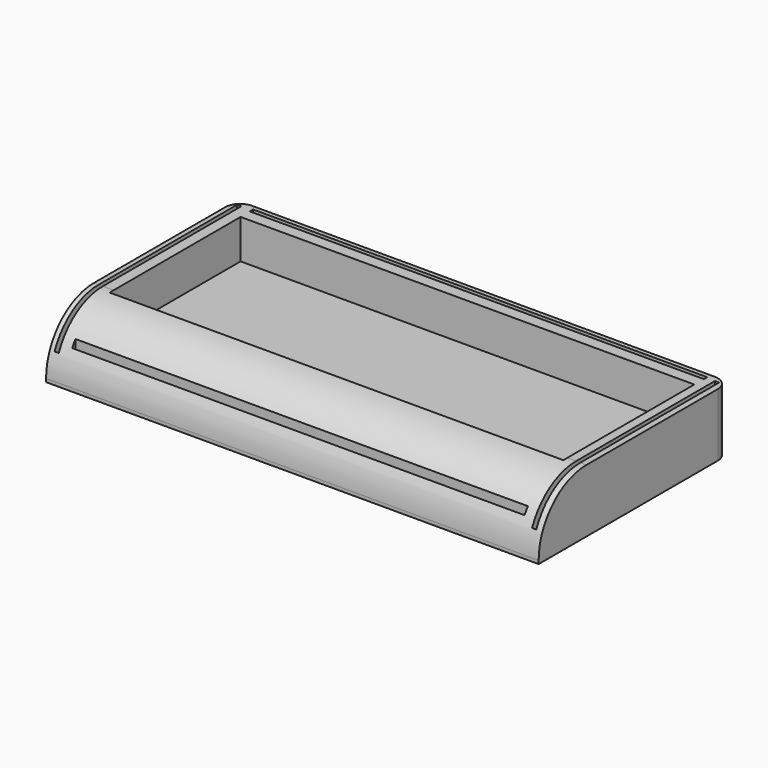
from build123d import *

# Parameters (mm, degrees)
F0_W        = 165
F0_H        = 80
F0_W_2      = 151.5524461865
F0_H_2      = 1.4
F0_W_3      = 1.4
F0_H_3      = 76.4191485941
F0_H_4      = 76.5563435853
F0_W_4      = 151.9825384021
F0_H_5      = 54.7616053373
F0_W_5      = 152.1170958877
F1_DEPTH    = 21.11
F2_T1_DEPTH = 265
F3_DEPTH    = 8
F4_R        = 5


# Not quite as in the source:
# - a fillet or chamfer that OpenCascade refuses, or shapes differently, is made with other operations: its cross-section is extruded or revolved along the edge and cut away or added


with BuildPart() as f1:
    # F0 (on Top) → F1 (new body)
    with BuildSketch(Plane.XY):
        with Locations((-0.5210009217, 2.8526327014)):
            Rectangle(F0_W, F0_H)
        with Locations((-0.6515718997, -33.7715006649)):
            Rectangle(F0_W_2, F0_H_2, mode=Mode.SUBTRACT)
        with Locations((-80.7459980965, 2.6404876262)):
            Rectangle(F0_W_3, F0_H_3, mode=Mode.SUBTRACT)
        with Locations((79.2265801907, 2.7090851218)):
            Rectangle(F0_W_3, F0_H_4, mode=Mode.SUBTRACT)
        with Locations((-0.4365257919, 8.6810430512)):
            Rectangle(F0_W_4, F0_H_5, mode=Mode.SUBTRACT)
        with Locations((-0.4392154515, 40.7097370148)):
            Rectangle(F0_W_5, F0_H_2, mode=Mode.SUBTRACT)
    extrude(amount=F1_DEPTH)

    # F2: fillet of radius 20 on 1 edges, made by hand

    # F2_s2 → F2_t1 (cut)
    with BuildSketch(Plane.YZ.offset(-133.0210009217)):
        with BuildLine():
            ThreePointArc((-37.1473672986, 1.11), (-31.2895029223, 15.2521356237), (-17.1473672986, 21.11))
            Line((-17.1473672986, 21.11), (-37.1473672986, 21.11))
            Line((-37.1473672986, 21.11), (-37.1473672986, 1.11))
        make_face()
    extrude(amount=F2_T1_DEPTH, mode=Mode.SUBTRACT)

    # F0 (on Top) → F3 (join)
    with BuildSketch(Plane.XY):
        with Locations((-0.4365257919, 8.6810430512)):
            Rectangle(F0_W_4, F0_H_5)
    extrude(amount=F3_DEPTH)

    # F4
    f4_edges = [f1.edges().sort_by_distance(p)[0] for p in [
        (-83.021001, 42.852633, 10.555),
        (81.978999, 42.852633, 10.555),
    ]]
    fillet(f4_edges, radius=F4_R)


solid = f1.part
